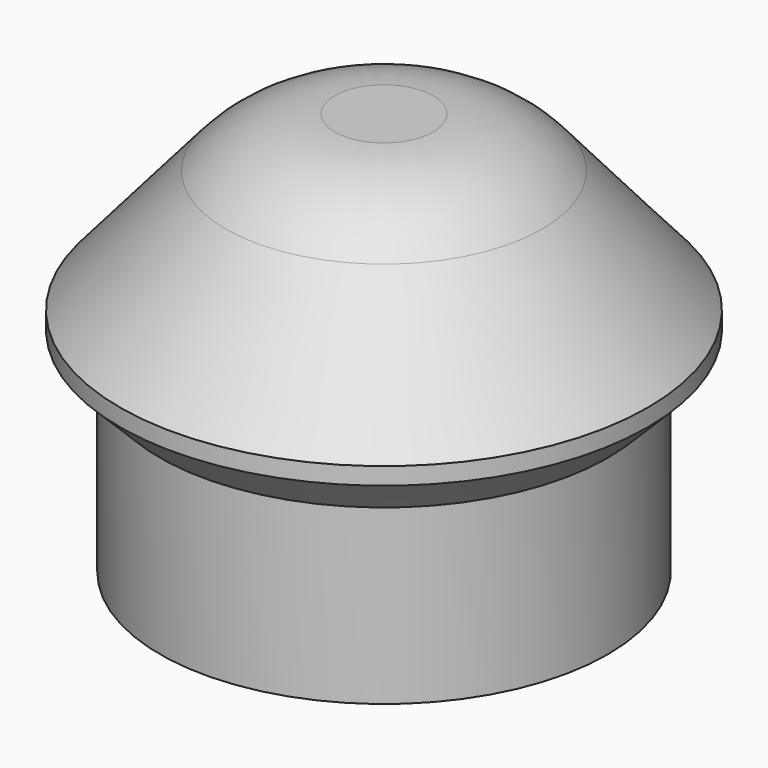
from build123d import *

# Parameters (mm, degrees)
F0_R        = 3.89
F1_DEPTH    = 3
F2_R        = 4.585
F2_R_2      = 3.89
F5_DEPTH    = 1
F5_FACE_R   = 4.585
F4_R        = 2
F7_R        = 2.5
F8_S5_R     = 3.89
F8_T6_DEPTH = 8


# Not quite as in the source:
# - a fillet or chamfer that OpenCascade refuses, or shapes differently, is made with other operations: its cross-section is extruded or revolved along the edge and cut away or added


with BuildPart() as f1:
    # F0 (on Top) → F1 (new body)
    with BuildSketch(Plane.XY):
        Circle(F0_R)
    extrude(amount=F1_DEPTH)

    # F2 (on face) → F5 (join)
    with BuildSketch(Plane.XY.offset(3)):
        Circle(F2_R)
        Circle(F2_R_2, mode=Mode.SUBTRACT)
        Circle(F2_R_2)
    extrude(amount=F5_DEPTH)

    # F5_face (on face) → F6 section 0
    with BuildSketch(Plane.XY.offset(4)):
        Circle(F5_FACE_R)
    # F4 (on offset) → F6 section 1
    with BuildSketch(Plane.XY.offset(7)):
        Circle(F4_R)
    loft()

    # F7
    f7_edges = [f1.edges().sort_by_distance(p)[0] for p in [
        (-2, 0, 7),
    ]]
    fillet(f7_edges, radius=F7_R)

    # F8: chamfer of 0.7 on 1 edges, made by hand


with BuildPart() as f8_tool2:
    # F8_s3 → F8_t4 (revolve)
    with BuildSketch(Plane.XZ):
        Polygon((4.585, 3.7), (3.885, 3), (4.585, 3), align=None)
    revolve(axis=Axis((0, 0, 3), (0, 0, 1)))

    # F8_s5 → F8_t6 (cut, symmetric)
    with BuildSketch(Plane.XY.offset(3.4)):
        Circle(F8_S5_R)
    extrude(amount=F8_T6_DEPTH, both=True, mode=Mode.SUBTRACT)


with BuildPart() as f1_1:
    add(f1.part)

    # F8_t1: cut F8_tool2
    add(f8_tool2.part, mode=Mode.SUBTRACT)


solid = f1_1.part
